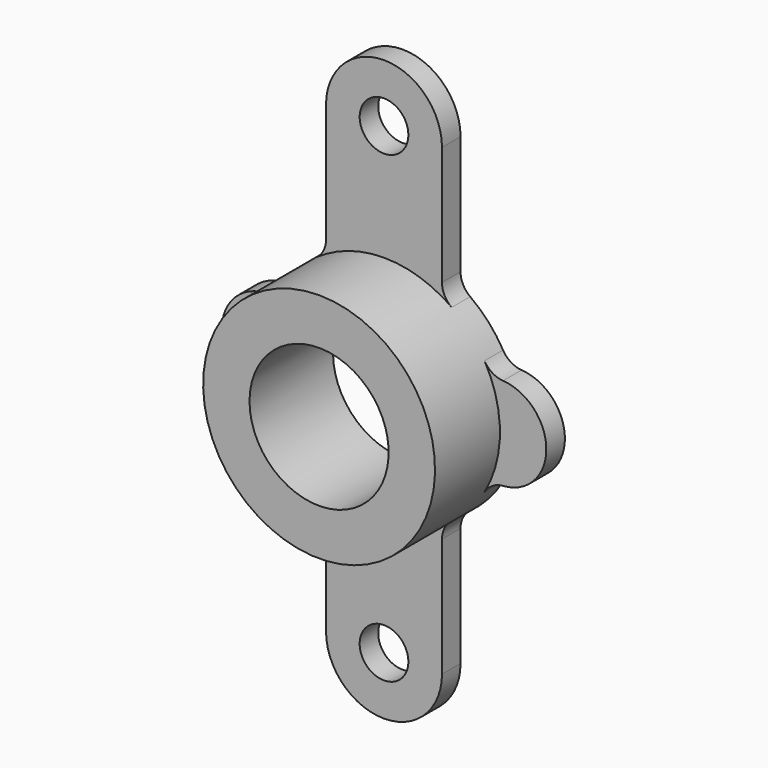
from build123d import *

# Parameters (mm, degrees)
F0_W        = 4.5
F0_H        = 5
F3_DEPTH    = 1
F4_W        = 10
F4_H        = 4
F5_DEPTH    = 1
F6_T1_DEPTH = 1
F7_R        = 3
F8_DEPTH    = 4.501


# Not quite as in the source:
# - a fillet or chamfer that OpenCascade refuses, or shapes differently, is made with other operations: its cross-section is extruded or revolved along the edge and cut away or added


with BuildPart() as f1:
    # F0 (on Right) → F1 (revolve)
    with BuildSketch(Plane.YZ):
        with Locations((-2.25, 2.5)):
            Rectangle(F0_W, F0_H)
    revolve(axis=Axis((0, -2.25, 0), (0, -1, 0)))

    # F2 (on face) → F3 (join)
    with BuildSketch(Plane(origin=(0, 0, 0), x_dir=(-1, 0, 0), z_dir=(0, 1, 0))):
        with BuildLine():
            ThreePointArc((-2.5, -10), (0, -12.5), (2.5, -10))
            Line((2.5, -10), (1.05, -10))
            ThreePointArc((1.05, -10), (0, -11.05), (-1.05, -10))
            Line((-1.05, -10), (-2.5, -10))
        make_face()
        with BuildLine():
            Line((1.05, -10), (2.5, -10))
            Line((2.5, -10), (2.5, 10))
            Line((2.5, 10), (1.05, 10))
            ThreePointArc((1.05, 10), (0, 8.95), (-1.05, 10))
            Line((-1.05, 10), (-2.5, 10))
            Line((-2.5, 10), (-2.5, -10))
            Line((-2.5, -10), (-1.05, -10))
            ThreePointArc((-1.05, -10), (0, -8.95), (1.05, -10))
        make_face()
        with BuildLine():
            Line((1.05, 10), (2.5, 10))
            ThreePointArc((2.5, 10), (0, 12.5), (-2.5, 10))
            Line((-2.5, 10), (-1.05, 10))
            ThreePointArc((-1.05, 10), (0, 11.05), (1.05, 10))
        make_face()
    extrude(amount=-F3_DEPTH)

    # F4 (on face) → F5 (join)
    with BuildSketch(Plane(origin=(0, 0, 0), x_dir=(-1, 0, 0), z_dir=(0, 1, 0))):
        Rectangle(F4_W, F4_H)
        with BuildLine():
            Line((5, 2), (5, -2))
            ThreePointArc((5, -2), (7, 0), (5, 2))
        make_face()
        with BuildLine():
            ThreePointArc((-5, 2), (-7, 0), (-5, -2))
            Line((-5, -2), (-5, 2))
        make_face()
    extrude(amount=-F5_DEPTH)

    # F6: fillet of radius 1 on 8 edges, made by hand

    # F6_s2 → F6_t1 (join)
    with BuildSketch(Plane.XZ):
        with BuildLine():
            ThreePointArc((-2.5, 4.8733971724), (-2.610243479, 4.4169617078), (-2.9166666667, 4.0611643103))
            ThreePointArc((-2.9166666667, 4.0611643103), (-2.7116700904, 4.2008148401), (-2.5, 4.3301270189))
            Line((-2.5, 4.3301270189), (-2.5, 4.8733971724))
        make_face()
        with BuildLine():
            ThreePointArc((-2.9166666667, -4.0611643103), (-2.610243479, -4.4169617078), (-2.5, -4.8733971724))
            Line((-2.5, -4.8733971724), (-2.5, -4.3301270189))
            ThreePointArc((-2.5, -4.3301270189), (-2.7116700904, -4.2008148401), (-2.9166666667, -4.0611643103))
        make_face()
        with BuildLine():
            ThreePointArc((4.3333333333, 2.4944382578), (4.6708497378, 2.144797772), (5.1333333333, 1.9955506063))
            Line((5.1333333333, 1.9955506063), (5.1266666667, 1.895773076))
            ThreePointArc((5.1266666667, 1.895773076), (5, 1.9), (4.582575695, 1.9))
            Line((4.582575695, 1.9), (4.4909241811, 1.96))
            ThreePointArc((4.4909241811, 1.96), (4.3755080286, 2.2056585166), (4.2466666667, 2.4445494927))
            Line((4.2466666667, 2.4445494927), (4.3333333333, 2.4944382578))
        make_face()
        with BuildLine():
            ThreePointArc((-4.3333333333, 2.4944382578), (-4.6708497378, 2.144797772), (-5.1333333333, 1.9955506063))
            Line((-5.1333333333, 1.9955506063), (-5.1266666667, 1.895773076))
            ThreePointArc((-5.1266666667, 1.895773076), (-5, 1.9), (-4.582575695, 1.9))
            Line((-4.582575695, 1.9), (-4.4909241811, 1.96))
            ThreePointArc((-4.4909241811, 1.96), (-4.3755080286, 2.2056585166), (-4.2466666667, 2.4445494927))
            Line((-4.2466666667, 2.4445494927), (-4.3333333333, 2.4944382578))
        make_face()
        with BuildLine():
            ThreePointArc((4.3333333333, -2.4944382578), (4.6708497378, -2.144797772), (5.1333333333, -1.9955506063))
            Line((5.1333333333, -1.9955506063), (5.1266666667, -1.895773076))
            ThreePointArc((5.1266666667, -1.895773076), (5, -1.9), (4.582575695, -1.9))
            Line((4.582575695, -1.9), (4.4909241811, -1.96))
            ThreePointArc((4.4909241811, -1.96), (4.3755080286, -2.2056585166), (4.2466666667, -2.4445494927))
            Line((4.2466666667, -2.4445494927), (4.3333333333, -2.4944382578))
        make_face()
        with BuildLine():
            ThreePointArc((-4.3333333333, -2.4944382578), (-4.6708497378, -2.144797772), (-5.1333333333, -1.9955506063))
            Line((-5.1333333333, -1.9955506063), (-5.1266666667, -1.895773076))
            ThreePointArc((-5.1266666667, -1.895773076), (-5, -1.9), (-4.582575695, -1.9))
            Line((-4.582575695, -1.9), (-4.4909241811, -1.96))
            ThreePointArc((-4.4909241811, -1.96), (-4.3755080286, -2.2056585166), (-4.2466666667, -2.4445494927))
            Line((-4.2466666667, -2.4445494927), (-4.3333333333, -2.4944382578))
        make_face()
        with BuildLine():
            ThreePointArc((2.9166666667, 4.0611643103), (2.610243479, 4.4169617078), (2.5, 4.8733971724))
            Line((2.5, 4.8733971724), (2.5, 4.3301270189))
            ThreePointArc((2.5, 4.3301270189), (2.7116700904, 4.2008148401), (2.9166666667, 4.0611643103))
        make_face()
        with BuildLine():
            ThreePointArc((2.9166666667, -4.0611643103), (2.610243479, -4.4169617078), (2.5, -4.8733971724))
            Line((2.5, -4.8733971724), (2.5, -4.3301270189))
            ThreePointArc((2.5, -4.3301270189), (2.7116700904, -4.2008148401), (2.9166666667, -4.0611643103))
        make_face()
    extrude(amount=F6_T1_DEPTH)

    # F7 (on face) → F8 (cut, through all)
    with BuildSketch(Plane(origin=(0, 0, 0), x_dir=(-1, 0, 0), z_dir=(0, 1, 0))):
        Circle(F7_R)
    extrude(amount=-F8_DEPTH, mode=Mode.SUBTRACT)


solid = f1.part
